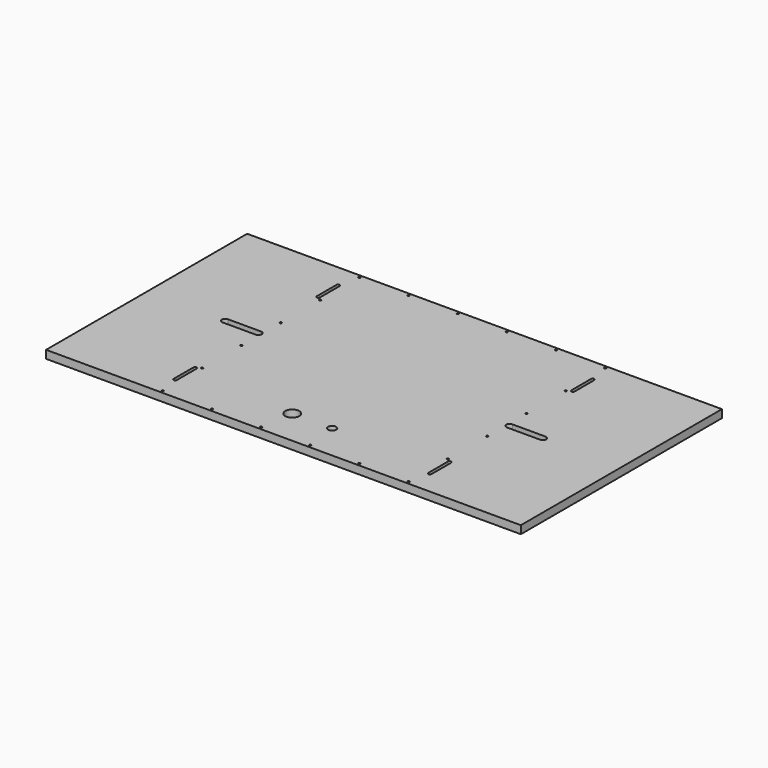
from build123d import *

# Parameters (mm, degrees)
F0_W             = 1190
F0_H             = 630
F1_DEPTH         = 20
F4_DEPTH         = 20.001
F4_COPIES2_COUNT = 2
F4_COPIES2_PITCH = 779.860552
F5_DEPTH         = 20.001
F7_R             = 17.515
F7_R_2           = 10.05
F8_DEPTH         = 20.001
F11_R            = 2.5
F12_DEPTH        = 20.001
F12_COPIES_COUNT = 4
F9_W             = 1190
F9_H             = 242.437693119
F13_DEPTH        = 20.001


# Not quite as in the source:
# - a pattern or mirror of a feature is missing from the dataset's text; its kind, count and spacing are read off the source's solid


with BuildPart() as f1:
    # F0 (on Top) → F1 (new body)
    with BuildSketch(Plane.XY):
        Rectangle(F0_W, F0_H)
    extrude(amount=F1_DEPTH)

    # F3 (on face) → F4 (cut, through all)
    with BuildSketch(Plane.XY.offset(20)):
        with BuildLine():
            Line((-323.2, 255), (-323.2, 193.2))
            ThreePointArc((-323.2, 193.2), (-319.1, 189.1), (-315, 193.2))
            Line((-315, 193.2), (-315, 255))
            ThreePointArc((-315, 255), (-319.1, 259.1), (-323.2, 255))
        make_face()
    f4 = extrude(amount=-F4_DEPTH, mode=Mode.SUBTRACT)

    # F4_copies: F4 across plane
    add(f4.mirror(Plane(origin=(0, 0, 0), x_dir=(0, 0, 1), z_dir=(1, 0, 0))), mode=Mode.SUBTRACT)

    # F4_copies1: F4 across plane
    add(f4.mirror(Plane(origin=(0, 0, 0), x_dir=(0, 0, -1), z_dir=(0, -1, 0))), mode=Mode.SUBTRACT)

    # F4_copies2: F4 ×2
    with Locations(*[Vector(0.818351433, -0.5747181327, 0) * (i * F4_COPIES2_PITCH) for i in range(1, F4_COPIES2_COUNT)]):
        add(f4, mode=Mode.SUBTRACT)

    # F3 (on face) → F5 (cut, through all)
    with BuildSketch(Plane.XY.offset(20)):
        with BuildLine():
            Line((-398, -8.5), (-315, -8.5))
            ThreePointArc((-315, -8.5), (-306.5, 0), (-315, 8.5))
            Line((-315, 8.5), (-398, 8.5))
            ThreePointArc((-398, 8.5), (-406.5, 0), (-398, -8.5))
        make_face()
    f5 = extrude(amount=-F5_DEPTH, mode=Mode.SUBTRACT)

    # F5_copies: F5 across plane
    add(f5.mirror(Plane(origin=(0, 0, 0), x_dir=(0, 0, 1), z_dir=(1, 0, 0))), mode=Mode.SUBTRACT)

    # F7 (on face) → F8 (cut, through all)
    with BuildSketch(Plane.XY.offset(20)):
        with Locations((-50, -225)):
            Circle(F7_R)
        with Locations((50, -225)):
            Circle(F7_R_2)
    extrude(amount=-F8_DEPTH, mode=Mode.SUBTRACT)

    # F11 (on face) → F12 (cut, through all)
    with BuildSketch(Plane.XY.offset(20)):
        with Locations((-308, 308)):
            Circle(F11_R)
        with Locations((-184.8, 308)):
            Circle(F11_R)
        with Locations((-61.6, 308)):
            Circle(F11_R)
        with Locations((61.6, 308)):
            Circle(F11_R)
        with Locations((184.8, 308)):
            Circle(F11_R)
        with Locations((308, 308)):
            Circle(F11_R)
    f12 = extrude(amount=-F12_DEPTH, mode=Mode.SUBTRACT)

    # F12_copies: F12 ×4 about axis
    f12_copies_axis = Axis((0, 0, 0), (0, 0, 1))
    for i in range(1, F12_COPIES_COUNT):
        add(f12.rotate(f12_copies_axis, i * 360 / F12_COPIES_COUNT), mode=Mode.SUBTRACT)

    # F9 (on face) → F13 (cut, through all)
    with BuildSketch(Plane.XY.offset(20)):
        with Locations((0, 436.2188465595)):
            Rectangle(F9_W, F9_H)
    extrude(amount=-F13_DEPTH, mode=Mode.SUBTRACT)


solid = f1.part
